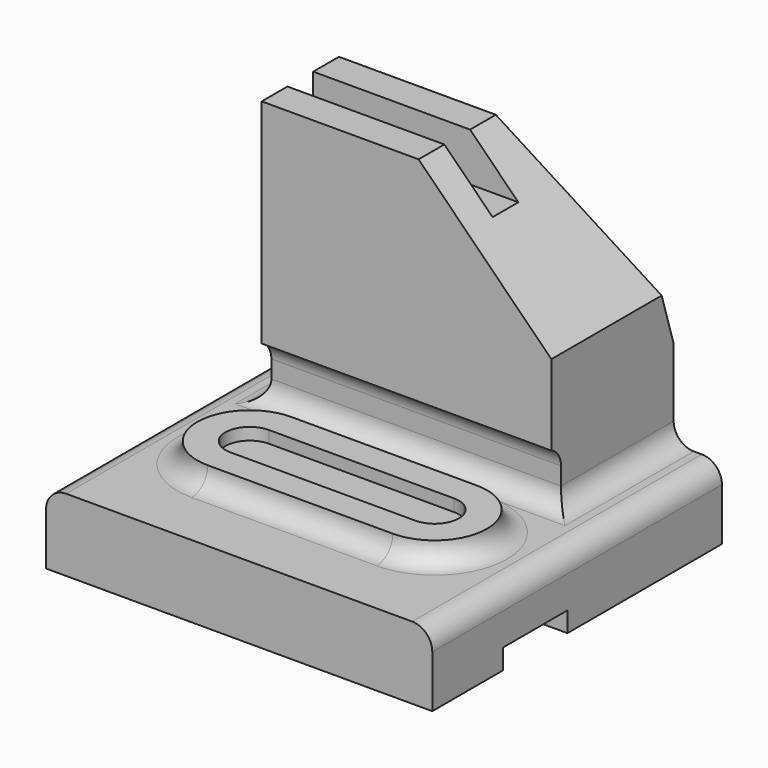
from build123d import *

# Parameters (mm, degrees)
F0_W          = 96
F0_H          = 90
F1_DEPTH      = 18
F2_W          = 72
F2_H          = 38
F4_DEPTH      = 67
F6_DEPTH      = 38.4
F7_W          = 8
F7_H          = 12
F8_DEPTH      = 71
F10_DEPTH     = 143.3
F11_W         = 20
F11_H         = 5
F12_DEPTH     = 107.3
F13_W         = 46
F13_H         = 26
F14_DEPTH     = 5
F15_W         = 46
F15_H         = 12
F16_DEPTH     = 3
F17_W         = 3
F17_H         = 14
F18_DEPTH     = 78.3
F19_T1_DEPTH  = 72
F19_T3_DEPTH  = 35
F19_T5_DEPTH  = 46
F19_T8_ANGLE  = 180
F19_T10_ANGLE = 180
F19_T15_DEPTH = 47.5
F19_T19_DEPTH = 84.5
F19_T27_DEPTH = 47.5
F19_T31_DEPTH = 84.5
F19_T35_DEPTH = 115


# Not quite as in the source:
# - a fillet or chamfer that OpenCascade refuses, or shapes differently, is made with other operations: its cross-section is extruded or revolved along the edge and cut away or added


with BuildPart() as f1:
    # F0 (on Top) → F1 (new body)
    with BuildSketch(Plane.XY):
        with Locations((48, 45)):
            Rectangle(F0_W, F0_H)
    extrude(amount=F1_DEPTH)

    # F2 (on face) → F4 (join, through all)
    with BuildSketch(Plane.XY.offset(18)):
        with Locations((48, 71)):
            Rectangle(F2_W, F2_H)
    extrude(amount=F4_DEPTH)

    # F5 (on face) → F6 (cut)
    with BuildSketch(Plane.XZ.offset(-52)):
        Polygon((84, 52), (84, 85), (51, 85), align=None)
    extrude(amount=-F6_DEPTH, mode=Mode.SUBTRACT)

    # F7 (on face) → F8 (cut)
    with BuildSketch(Plane(origin=(12, 0, 0), x_dir=(0, -1, 0), z_dir=(-1, 0, 0))):
        with Locations((-64, 79)):
            Rectangle(F7_W, F7_H)
    extrude(amount=-F8_DEPTH, mode=Mode.SUBTRACT)

    # F9 (on face) → F10 (cut)
    with BuildSketch(Plane(origin=(12, 0, 0), x_dir=(0, -1, 0), z_dir=(-1, 0, 0))):
        Polygon((-90, 40), (-76, 85), (-90, 85), align=None)
    extrude(amount=-F10_DEPTH, mode=Mode.SUBTRACT)

    # F11 (on face) → F12 (cut)
    with BuildSketch(Plane.YZ.offset(96)):
        with Locations((32, 2.5)):
            Rectangle(F11_W, F11_H)
    extrude(amount=-F12_DEPTH, mode=Mode.SUBTRACT)

    # F13 (on face) → F14 (join)
    with BuildSketch(Plane.XY.offset(18)):
        with BuildLine():
            Line((25, 18.9999999999), (25, 44.9999999999))
            ThreePointArc((25, 44.9999999999), (12, 31.9999999999), (25, 18.9999999999))
        make_face()
        with BuildLine():
            ThreePointArc((71, 18.9999999999), (84, 31.9999999999), (71, 44.9999999999))
            Line((71, 44.9999999999), (71, 18.9999999999))
        make_face()
        with Locations((48, 31.9999999999)):
            Rectangle(F13_W, F13_H)
    extrude(amount=F14_DEPTH)

    # F15 (on face) → F16 (cut)
    with BuildSketch(Plane.XY.offset(23)):
        with Locations((48, 31.9999999999)):
            Rectangle(F15_W, F15_H)
        with BuildLine():
            ThreePointArc((71, 25.9999999999), (77, 31.9999999999), (71, 37.9999999999))
            Line((71, 37.9999999999), (71, 25.9999999999))
        make_face()
        with BuildLine():
            Line((25, 25.9999999999), (25, 37.9999999999))
            ThreePointArc((25, 37.9999999999), (19, 31.9999999999), (25, 25.9999999999))
        make_face()
    extrude(amount=-F16_DEPTH, mode=Mode.SUBTRACT)

    # F17 (on face) → F18 (cut)
    with BuildSketch(Plane.YZ.offset(84)):
        with Locations((53.5, 25)):
            Rectangle(F17_W, F17_H)
    extrude(amount=-F18_DEPTH, mode=Mode.SUBTRACT)

    # F19: fillet of radius 5 on 10 edges, made by hand

    # F19_s2 → F19_t1 (join)
    with BuildSketch(Plane.YZ.offset(12)):
        with BuildLine():
            ThreePointArc((50, 18), (53.5355339059, 19.4644660941), (55, 23))
            Line((55, 23), (55, 18))
            Line((55, 18), (50, 18))
        make_face()
        with BuildLine():
            ThreePointArc((55, 27.417424305), (54.1833001327, 30.1560370926), (52, 32))
            Line((52, 32), (55, 32))
            Line((55, 32), (55, 27.417424305))
        make_face()
    extrude(amount=F19_T1_DEPTH)

    # F19_s4 → F19_t3 (join)
    with BuildSketch(Plane.XZ.offset(-90)):
        with BuildLine():
            ThreePointArc((89, 18), (85.4644660941, 19.4644660941), (84, 23))
            Line((84, 23), (84, 18))
            Line((84, 18), (89, 18))
        make_face()
        with BuildLine():
            ThreePointArc((7, 18), (10.5355339059, 19.4644660941), (12, 23))
            Line((12, 23), (12, 18))
            Line((12, 18), (7, 18))
        make_face()
    extrude(amount=F19_T3_DEPTH)

    # F19_s6 → F19_t5 (join)
    with BuildSketch(Plane.YZ.offset(25)):
        with BuildLine():
            ThreePointArc((13.9999999999, 18), (17.5355339058, 19.4644660941), (18.9999999999, 23))
            Line((18.9999999999, 23), (18.9999999999, 18))
            Line((18.9999999999, 18), (13.9999999999, 18))
        make_face()
        with BuildLine():
            ThreePointArc((49.9999999999, 18), (46.464466094, 19.4644660941), (44.9999999999, 23))
            Line((44.9999999999, 23), (44.9999999999, 18))
            Line((44.9999999999, 18), (49.9999999999, 18))
        make_face()
    extrude(amount=F19_T5_DEPTH)

    # F19_s7 → F19_t8 (revolve)
    with BuildSketch(Plane.YZ.offset(25)):
        with BuildLine():
            ThreePointArc((49.9999999999, 18), (46.464466094, 19.4644660941), (44.9999999999, 23))
            Line((44.9999999999, 23), (44.9999999999, 18))
            Line((44.9999999999, 18), (49.9999999999, 18))
        make_face()
    revolve(axis=Axis((25, 31.9999999999, 18), (0, 0, 1)), revolution_arc=F19_T8_ANGLE)

    # F19_s9 → F19_t10 (revolve)
    with BuildSketch(Plane.YZ.offset(71)):
        with BuildLine():
            ThreePointArc((13.9999999999, 18), (17.5355339058, 19.4644660941), (18.9999999999, 23))
            Line((18.9999999999, 23), (18.9999999999, 18))
            Line((18.9999999999, 18), (13.9999999999, 18))
        make_face()
    revolve(axis=Axis((71, 31.9999999999, 18), (0, 0, 1)), revolution_arc=F19_T10_ANGLE)


with BuildPart() as f19_tool13:
    # F19_s14 → F19_t15 (new body)
    with BuildSketch(Plane.XZ.offset(-42.5)):
        with BuildLine():
            ThreePointArc((89, 18), (85.4644660941, 19.4644660941), (84, 23))
            Line((84, 23), (84, 18))
            Line((84, 18), (89, 18))
        make_face()
    extrude(amount=-F19_T15_DEPTH)

    split(bisect_by=Plane.XZ.offset(-55), keep=Keep.TOP)


with BuildPart() as f19_tool17:
    # F19_s18 → F19_t19 (new body)
    with BuildSketch(Plane.YZ.offset(96.5)):
        with BuildLine():
            ThreePointArc((50, 18), (53.5355339059, 19.4644660941), (55, 23))
            Line((55, 23), (55, 18))
            Line((55, 18), (50, 18))
        make_face()
    extrude(amount=-F19_T19_DEPTH)

    split(bisect_by=Plane.YZ.offset(96), keep=Keep.BOTTOM)

    split(bisect_by=Plane.YZ.offset(84), keep=Keep.TOP)


with BuildPart() as f19_tool13_1:
    add(f19_tool13.part)

    # F19_t22: intersect F19_tool17
    add(f19_tool17.part, mode=Mode.INTERSECT)


with BuildPart() as f1_1:
    add(f1.part)

    # F19_t11: union F19_tool13
    add(f19_tool13_1.part)


with BuildPart() as f19_tool25:
    # F19_s26 → F19_t27 (new body)
    with BuildSketch(Plane.XZ.offset(-90)):
        with BuildLine():
            ThreePointArc((7, 18), (10.5355339059, 19.4644660941), (12, 23))
            Line((12, 23), (12, 18))
            Line((12, 18), (7, 18))
        make_face()
    extrude(amount=F19_T27_DEPTH)

    split(bisect_by=Plane.XZ.offset(-55), keep=Keep.TOP)


with BuildPart() as f19_tool29:
    # F19_s30 → F19_t31 (new body)
    with BuildSketch(Plane.YZ.offset(84)):
        with BuildLine():
            ThreePointArc((50, 18), (53.5355339059, 19.4644660941), (55, 23))
            Line((55, 23), (55, 18))
            Line((55, 18), (50, 18))
        make_face()
    extrude(amount=-F19_T31_DEPTH)

    split(bisect_by=Plane.YZ, keep=Keep.TOP)

    split(bisect_by=Plane.YZ.offset(12), keep=Keep.BOTTOM)


with BuildPart() as f19_tool25_1:
    add(f19_tool25.part)

    # F19_t34: intersect F19_tool29
    add(f19_tool29.part, mode=Mode.INTERSECT)


with BuildPart() as f1_2:
    add(f1_1.part)

    # F19_t23: union F19_tool25
    add(f19_tool25_1.part)

    # F19_s36 → F19_t35 (cut)
    with BuildSketch(Plane.XZ.offset(-102.5)):
        with BuildLine():
            ThreePointArc((96, 13), (94.5355339059, 16.5355339059), (91, 18))
            Line((91, 18), (96, 18))
            Line((96, 18), (96, 13))
        make_face()
        with BuildLine():
            ThreePointArc((0, 13), (1.4644660941, 16.5355339059), (5, 18))
            Line((5, 18), (0, 18))
            Line((0, 18), (0, 13))
        make_face()
    extrude(amount=F19_T35_DEPTH, mode=Mode.SUBTRACT)


solid = f1_2.part
